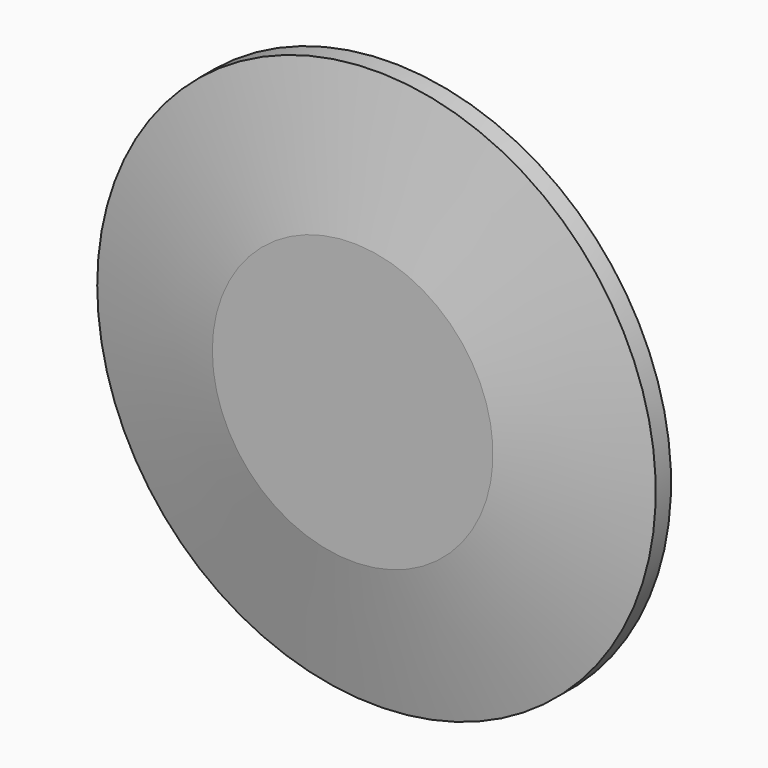
from build123d import *

# Parameters (mm, degrees)
F2_TEXT_SIZE = 11.9723744577
F3_DEPTH     = 1


# Not quite as in the source:
# - Text() gives the source's letters only with a copy of the font that has no kerning and outlines rounded to 1/6400 em; it was checked with that copy


with BuildPart() as f1:
    # F0 (on Top) → F1 (revolve)
    with BuildSketch(Plane.XY):
        Polygon((-54.7159127891, -6.557055291), (-7.056819275, -16.7727265507), (41.0760901868, -16.7727265507), (41.0760901868, -2.8636364732), (-32.0113636553, -2.8636364732), (-54.7159127891, 0), align=None)
    revolve(axis=Axis((41.0760901868, -9.8181815119, 0), (0, 1, 0)))

    # F2 (on face) → F3 (join)
    with BuildSketch(Plane(origin=(0, -2.8636364732, 0), x_dir=(-1, 0, 0), z_dir=(0, 1, 0))):
        with Locations((-113.98999355, -3.5863629458)):
            Text('Carter Is Da Best (Failure)', F2_TEXT_SIZE, font='Open Sans', font_style=FontStyle.BOLDITALIC, text_align=(TextAlign.LEFT, TextAlign.BOTTOM))
    extrude(amount=F3_DEPTH)


solid = f1.part
